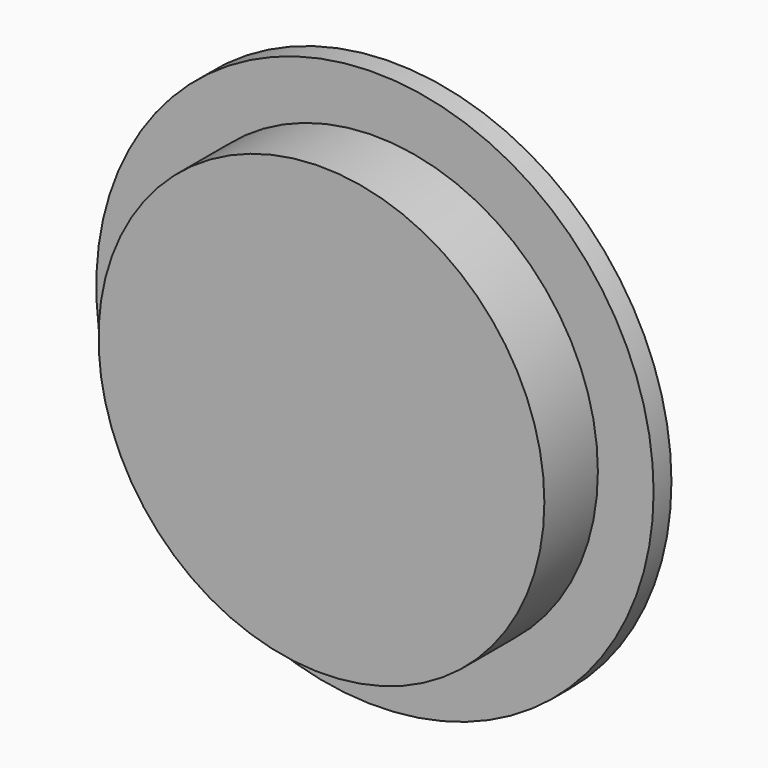
from build123d import *

# Parameters (mm, degrees)
F0_R      = 10
F1_DEPTH  = 3
F0_R_2    = 12.5
F1_FACE_R = 10
F2_DEPTH  = 1


# Not quite as in the source:
# - a feature of the source that left no trace in its solid (it failed there, or was rolled back) is left out


with BuildPart() as f1:
    # F0 (on Front) → F1 (new body)
    with BuildSketch(Plane.XZ):
        Circle(F0_R)
    extrude(amount=F1_DEPTH)

    # F0 (on Front) + F1_face (on face) → F2 (join)
    with BuildSketch(Plane.XZ):
        Circle(F0_R_2)
        Circle(F0_R, mode=Mode.SUBTRACT)
    with BuildSketch(Plane.XZ.offset(3)):
        Circle(F1_FACE_R)
    extrude(amount=F2_DEPTH)


solid = f1.part
